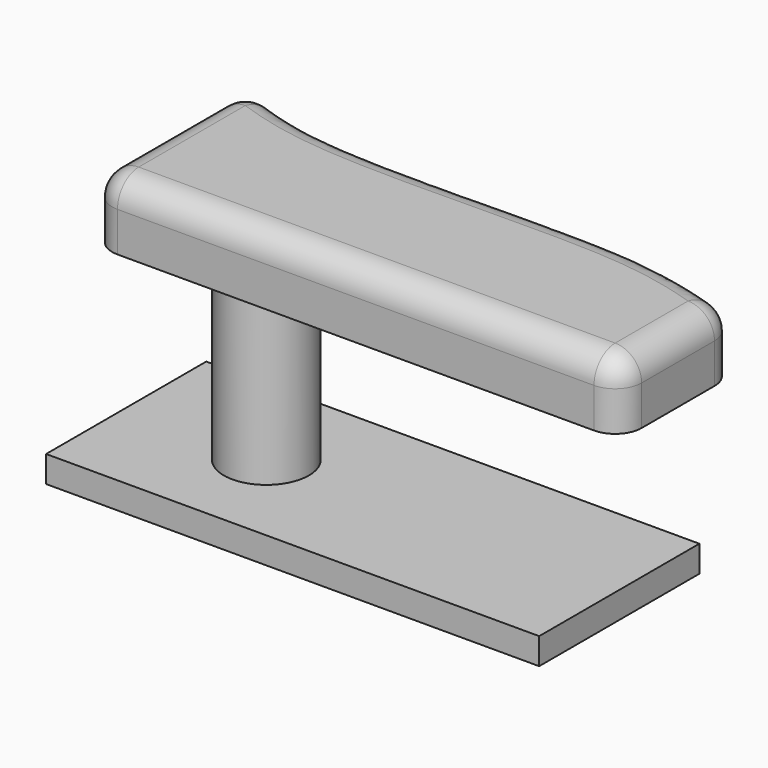
from build123d import *

# Parameters (mm, degrees)
F0_W     = 101.6
F0_H     = 38.1
F1_DEPTH = 12.7
F3_DEPTH = 25.4
F4_R     = 5.08
F5_R     = 8.1585403427
F6_DEPTH = 38.1
F7_W     = 94.6341231465
F7_H     = 38.4192988276
F8_DEPTH = 5.08


# Not quite as in the source:
# - two fillets or chamfers of one size are made in one step


with BuildPart() as f1:
    # F0 (on Top) → F1 (new body)
    with BuildSketch(Plane.XY):
        Rectangle(F0_W, F0_H)
    extrude(amount=F1_DEPTH)

    # F2 (on face) → F3 (cut)
    with BuildSketch(Plane.XY.offset(12.7)):
        with BuildLine():
            Line((-50.8, 29.4957049191), (-50.8, 19.05))
            add(Edge.make_bspline(
                [(-50.8, 19.05), (-44.8058190597, 16.5548569949), (-29.3022913601, 10.1013449841), (28.5345191575, 14.5340371651), (44.5678818935, 9.2526124329), (50.8, 7.199739106)],
                knots=[0, 0, 0, 0, 0.2781516974, 0.7194198154, 1, 1, 1, 1], degree=3))
            Line((50.8, 7.199739106), (51.4432899654, 29.4957049191))
            Line((51.4432899654, 29.4957049191), (-50.8, 29.4957049191))
        make_face()
    extrude(amount=-F3_DEPTH, mode=Mode.SUBTRACT)

    # F4
    f4_edges = [f1.edges().sort_by_distance(p)[0] for p in [
        (0, -19.05, 12.7),
        (50.8, -5.92513, 12.7),
        (-0.16927, 12.372824, 12.7),
        (-50.8, 0, 12.7),
        (-50.8, 19.05, 6.35),
        (-50.8, -19.05, 6.35),
        (50.8, 7.199739, 6.35),
        (50.8, -19.05, 6.35),
    ]]
    fillet(f4_edges, radius=F4_R)

    # F5 (on Top) → F6 (join)
    with BuildSketch(Plane.XY):
        with Locations((-32.3988236487, 0)):
            Circle(F5_R)
    extrude(amount=-F6_DEPTH)

    # F7 (on face) → F8 (join)
    with BuildSketch(Plane(origin=(0, 0, -38.1), x_dir=(1, 0, 0), z_dir=(0, 0, -1))):
        with Locations((-12.0352953672, -0.0617783517)):
            Rectangle(F7_W, F7_H)
    extrude(amount=F8_DEPTH)


solid = f1.part
